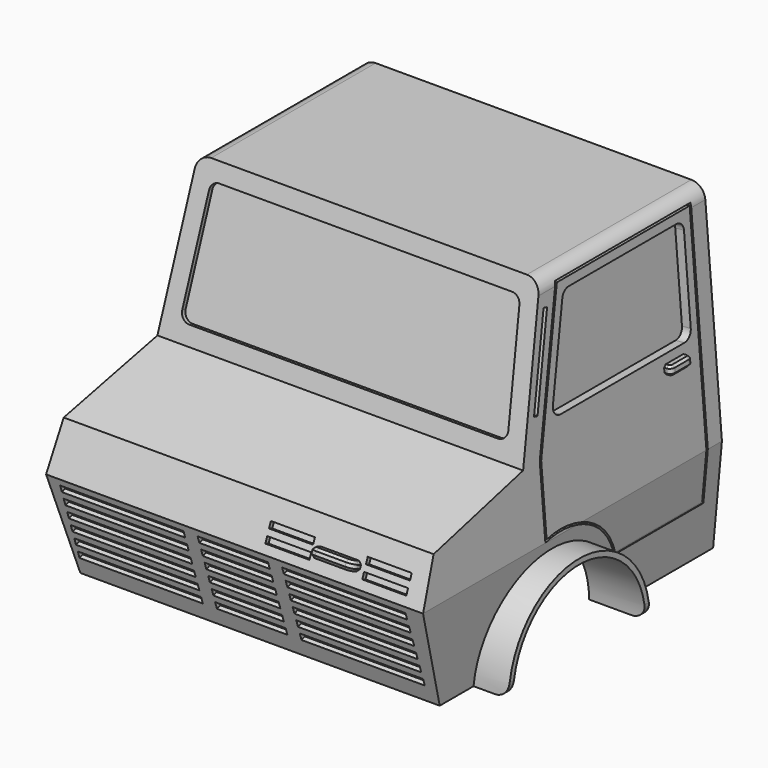
from build123d import *

# Parameters (mm, degrees)
F1_DEPTH       = 2140
F3_DEPTH       = 2500
F4_W           = 400
F4_H           = 40
F4_W_2         = 700
F5_DEPTH       = 25
F7_DEPTH       = 25
F9_DEPTH       = 50
F11_DEPTH      = 50
F13_DEPTH      = 150
F13_DEPTH_BACK = 2290
F14_T1_DEPTH   = 430
F14_T3_DEPTH   = 430
F14_T8_DEPTH   = 1536.0313143724
F14_T13_DEPTH  = 1536.0313143724
F14_T18_DEPTH  = 1536.0313143724
F14_T23_DEPTH  = 1536.0313143724
F14_T28_DEPTH  = 1536.0313143724
F14_T33_DEPTH  = 1536.0313143724
F15_W          = 1800
F15_H          = 1110
F15_H_2        = 10
F15_H_3        = 730
F16_DEPTH      = 200
F18_DEPTH      = 25
F19_W          = 150
F19_H          = 50
F20_DEPTH      = 40
F21_W          = 150
F21_H          = 50
F22_DEPTH      = 40
F23_R          = 25
F24_SIZE       = 12.5
F27_DEPTH      = 25
F28_W          = 250
F28_H          = 35
F29_DEPTH      = 25
F28_H_2        = 50
F30_DEPTH      = 60
F31_R          = 40
F32_SIZE       = 15
F33_DEPTH      = 25


# Not quite as in the source:
# - a fillet or chamfer that OpenCascade refuses, or shapes differently, is made with other operations: its cross-section is extruded or revolved along the edge and cut away or added
# - a feature names something its author has since deleted; it is built from what else it names


with BuildPart() as f1:
    # F0 (on Right) → F1 (new body)
    with BuildSketch(Plane.YZ):
        with BuildLine():
            Line((-868.0252010454, -338.8581766918), (-687.2093945233, -888.8581766918))
            Line((-687.2093945233, -888.8581766918), (-447.2093945233, -888.8581766918))
            ThreePointArc((-447.2093945233, -888.8581766918), (52.7906054767, -388.8581766918), (552.7906054767, -888.8581766918))
            Line((552.7906054767, -888.8581766918), (1252.7906054767, -888.8581766918))
            Line((1252.7906054767, -888.8581766918), (1252.7906054767, 911.1418233082))
            Line((1252.7906054767, 911.1418233082), (86.0372496318, 911.1418233082))
            Line((86.0372496318, 911.1418233082), (-118.0252010454, 61.1418233082))
            Line((-118.0252010454, 61.1418233082), (-768.0252010454, -88.8581766918))
            Line((-768.0252010454, -88.8581766918), (-868.0252010454, -338.8581766918))
        make_face()
    extrude(amount=F1_DEPTH)

    # F2 (on face) → F3 (cut)
    with BuildSketch(Plane(origin=(0, 1252.7906054767, 0), x_dir=(-1, 0, 0), z_dir=(0, 1, 0))):
        Polygon((-2140, 911.1418233082), (-2140, -338.8581766918), (-2040, 911.1418233082), align=None)
        Polygon((-2140, -338.8581766918), (-2140, -888.8581766918), (-2090, -888.8581766918), align=None)
        Polygon((0, -338.8581766918), (-50, -888.8581766918), (0, -888.8581766918), align=None)
        Polygon((-100, 911.1418233082), (0, -338.8581766918), (0, 911.1418233082), align=None)
    extrude(amount=-F3_DEPTH, mode=Mode.SUBTRACT)

    # F4 (on face) → F5 (cut)
    with BuildSketch(Plane(origin=(0, -883.8950331202, -290.5858059899), x_dir=(1, 0, 0), z_dir=(0, -0.9499797347, -0.3123115489))):
        with Locations((1050, -110.8141057509)):
            Rectangle(F4_W, F4_H)
        with Locations((1680, -110.8141057509)):
            Rectangle(F4_W_2, F4_H)
        with Locations((1680, -190.8141057509)):
            Rectangle(F4_W_2, F4_H)
        with Locations((1050, -190.8141057509)):
            Rectangle(F4_W, F4_H)
        with Locations((420, -190.8141057509)):
            Rectangle(F4_W_2, F4_H)
        with Locations((420, -110.8141057509)):
            Rectangle(F4_W_2, F4_H)
        with Locations((420, -270.8141057509)):
            Rectangle(F4_W_2, F4_H)
        with Locations((1050, -270.8141057509)):
            Rectangle(F4_W, F4_H)
        with Locations((1680, -270.8141057509)):
            Rectangle(F4_W_2, F4_H)
        with Locations((1680, -350.8141057509)):
            Rectangle(F4_W_2, F4_H)
        with Locations((1050, -350.8141057509)):
            Rectangle(F4_W, F4_H)
        with Locations((420, -350.8141057509)):
            Rectangle(F4_W_2, F4_H)
        with Locations((420, -430.8141057509)):
            Rectangle(F4_W_2, F4_H)
        with Locations((1050, -430.8141057509)):
            Rectangle(F4_W, F4_H)
        with Locations((1680, -430.8141057509)):
            Rectangle(F4_W_2, F4_H)
        with Locations((1050, -510.8141057509)):
            Rectangle(F4_W, F4_H)
        with Locations((1680, -510.8141057509)):
            Rectangle(F4_W_2, F4_H)
        with Locations((420, -510.8141057509)):
            Rectangle(F4_W_2, F4_H)
    extrude(amount=-F5_DEPTH, mode=Mode.SUBTRACT)

    # F6 (on face) → F7 (cut)
    with BuildSketch(Plane(origin=(0, -125.4721115769, 30.1225253883), x_dir=(1, 0, 0), z_dir=(0, -0.9723710875, 0.2334405025))):
        with BuildLine():
            ThreePointArc((238.7847050975, 806.0525443848), (204.8280302743, 792.7532832732), (188.9353028494, 759.9303137829))
            Line((188.9353028494, 759.9303137829), (144.2722089495, 185.7784483863))
            ThreePointArc((144.2722089495, 185.7784483863), (157.4208723093, 147.944004165), (194.1216111976, 131.9006789882))
            Line((194.1216111976, 131.9006789882), (1945.8783888024, 131.9006789882))
            ThreePointArc((1945.8783888024, 131.9006789882), (1982.5791276907, 147.944004165), (1995.7277910505, 185.7784483863))
            Line((1995.7277910505, 185.7784483863), (1951.0646971506, 759.9303137829))
            ThreePointArc((1951.0646971506, 759.9303137829), (1935.1719697257, 792.7532832732), (1901.2152949025, 806.0525443848))
            Line((1901.2152949025, 806.0525443848), (238.7847050975, 806.0525443848))
        make_face()
    extrude(amount=-F7_DEPTH, mode=Mode.SUBTRACT)

    # F8 (on face) → F9 (cut)
    with BuildSketch(Plane(origin=(2099.4548349212, 0, 167.9563867937), x_dir=(0, 1, 0), z_dir=(0.9968152785, 0, 0.0797452223))):
        with BuildLine():
            Line((1152.7906054767, -508.4337834687), (1152.7906054767, 695.5598369298))
            Line((1152.7906054767, 695.5598369298), (192.4028323197, 695.5598369298))
            Line((192.4028323197, 695.5598369298), (0, -108.4337834687))
            Line((0, -108.4337834687), (0, -508.4337834687))
            ThreePointArc((0, -508.4337834687), (111.5695780666, -493.7074634076), (223.1391561332, -508.4337834687))
            Line((223.1391561332, -508.4337834687), (256.9923092676, -508.4337834687))
            ThreePointArc((256.9923092676, -508.4337834687), (134.4170810173, -484.3010551602), (10, -495.5910997734))
            Line((10, -495.5910997734), (10, -109.6136704941))
            Line((10, -109.6136704941), (200.2921007484, 685.5598369298))
            Line((200.2921007484, 685.5598369298), (1142.7906054767, 685.5598369298))
            Line((1142.7906054767, 685.5598369298), (1142.7906054767, -508.4337834687))
            Line((1142.7906054767, -508.4337834687), (1152.7906054767, -508.4337834687))
        make_face()
        with BuildLine():
            Line((1152.7906054767, -782.6949255494), (1152.7906054767, -508.4337834687))
            Line((1152.7906054767, -508.4337834687), (1142.7906054767, -508.4337834687))
            Line((1142.7906054767, -508.4337834687), (1142.7906054767, -772.6949255494))
            Line((1142.7906054767, -772.6949255494), (524.8433534379, -772.6949255494))
            ThreePointArc((524.8433534379, -772.6949255494), (420.590506836, -610.4885853327), (256.9923092676, -508.4337834687))
            Line((256.9923092676, -508.4337834687), (223.1391561332, -508.4337834687))
            ThreePointArc((223.1391561332, -508.4337834687), (404.5398026813, -608.9560575502), (517.7905329259, -782.6949255494))
            Line((517.7905329259, -782.6949255494), (1152.7906054767, -782.6949255494))
        make_face()
        with BuildLine():
            ThreePointArc((1092.7906054767, 585.5598369298), (1078.145944536, 620.9151759891), (1042.7906054767, 635.5598369298))
            Line((1042.7906054767, 635.5598369298), (279.1847850354, 635.5598369298))
            ThreePointArc((279.1847850354, 635.5598369298), (248.215796316, 624.8144129394), (230.5578041703, 597.1967064375))
            Line((230.5578041703, 597.1967064375), (115.6895301314, 117.1967064375))
            ThreePointArc((115.6895301314, 117.1967064375), (125.061934987, 74.5908482103), (164.3165109966, 55.5598369298))
            Line((164.3165109966, 55.5598369298), (1042.7906054767, 55.5598369298))
            ThreePointArc((1042.7906054767, 55.5598369298), (1078.145944536, 70.2044978704), (1092.7906054767, 105.5598369298))
            Line((1092.7906054767, 105.5598369298), (1092.7906054767, 585.5598369298))
        make_face()
    extrude(amount=-F9_DEPTH, mode=Mode.SUBTRACT)

    # F10 (on face) → F11 (cut)
    with BuildSketch(Plane(origin=(26.9362620582, 0, -2.1549009647), x_dir=(0, -1, 0), z_dir=(-0.9968152785, 0, 0.0797452223))):
        with BuildLine():
            Line((-1152.7906054767, -612.040149864), (-517.7376456074, -612.040149864))
            ThreePointArc((-517.7376456074, -612.040149864), (-312.7747219376, -373.0527728554), (0.0839169816, -337.7790077833))
            Line((0.0839169816, -337.7790077833), (0.0839169816, 62.2209922167))
            Line((0.0839169816, 62.2209922167), (-192.318915338, 866.2146126152))
            Line((-192.318915338, 866.2146126152), (-1152.7906054767, 866.2146126152))
            Line((-1152.7906054767, 866.2146126152), (-1152.7906054767, -612.040149864))
        make_face()
        with BuildLine():
            Line((-1142.7906054767, -602.040149864), (-1142.7906054767, 856.2146126152))
            Line((-1142.7906054767, 856.2146126152), (-200.2081837667, 856.2146126152))
            Line((-200.2081837667, 856.2146126152), (-9.9160830184, 61.0411051913))
            Line((-9.9160830184, 61.0411051913), (-9.9160830184, -324.9354323363))
            ThreePointArc((-9.9160830184, -324.9354323363), (-320.0389671232, -365.5952501122), (-524.7906054767, -602.040149864))
            Line((-524.7906054767, -602.040149864), (-1142.7906054767, -602.040149864))
        make_face(mode=Mode.SUBTRACT)
        with BuildLine():
            ThreePointArc((-1042.7906054767, 806.2146126152), (-1078.145944536, 791.5699516745), (-1092.7906054767, 756.2146126152))
            Line((-1092.7906054767, 756.2146126152), (-1092.7906054767, 276.2146126152))
            ThreePointArc((-1092.7906054767, 276.2146126152), (-1078.145944536, 240.8592735558), (-1042.7906054767, 226.2146126152))
            Line((-1042.7906054767, 226.2146126152), (-164.2325940149, 226.2146126152))
            ThreePointArc((-164.2325940149, 226.2146126152), (-124.9780180054, 245.2456238957), (-115.6056131498, 287.8514821229))
            Line((-115.6056131498, 287.8514821229), (-230.4738871887, 767.8514821229))
            ThreePointArc((-230.4738871887, 767.8514821229), (-248.1318793343, 795.4691886247), (-279.1008680538, 806.2146126152))
            Line((-279.1008680538, 806.2146126152), (-1042.7906054767, 806.2146126152))
        make_face()
    extrude(amount=-F11_DEPTH, mode=Mode.SUBTRACT)

    # F12 (on Right) → F13 (join, two sides)
    with BuildSketch(Plane.YZ) as f13_sk:
        with BuildLine():
            Line((522.7906054767, -888.8581766918), (552.7906054767, -888.8581766918))
            ThreePointArc((552.7906054767, -888.8581766918), (52.7906054767, -388.8581766918), (-447.2093945233, -888.8581766918))
            Line((-447.2093945233, -888.8581766918), (-417.2093945233, -888.8581766918))
            ThreePointArc((-417.2093945233, -888.8581766918), (52.7906054767, -418.8581773039), (522.7906054767, -888.8581766918))
        make_face()
    extrude(amount=-F13_DEPTH)
    extrude(f13_sk.sketch, amount=F13_DEPTH_BACK)

    # F14: fillet of radius 80 on 6 edges, made by hand

    # F14_s2 → F14_t1 (cut)
    with BuildSketch(Plane.XZ.offset(217.2093945233)):
        with BuildLine():
            ThreePointArc((-70, -888.8581766918), (-126.5685424949, -865.4267191867), (-150, -808.8581766918))
            Line((-150, -808.8581766918), (-150, -888.8581766918))
            Line((-150, -888.8581766918), (-70, -888.8581766918))
        make_face()
        with BuildLine():
            ThreePointArc((2210, -888.8581766918), (2266.5685424949, -865.4267191867), (2290, -808.8581766918))
            Line((2290, -808.8581766918), (2290, -888.8581766918))
            Line((2290, -888.8581766918), (2210, -888.8581766918))
        make_face()
    extrude(amount=F14_T1_DEPTH, mode=Mode.SUBTRACT)

    # F14_s4 → F14_t3 (cut)
    with BuildSketch(Plane.XZ.offset(-752.7906054767)):
        with BuildLine():
            ThreePointArc((-150, -808.8581766918), (-126.5685424949, -865.4267191867), (-70, -888.8581766918))
            Line((-70, -888.8581766918), (-150, -888.8581766918))
            Line((-150, -888.8581766918), (-150, -808.8581766918))
        make_face()
        with BuildLine():
            ThreePointArc((2290, -808.8581766918), (2266.5685424949, -865.4267191867), (2210, -888.8581766918))
            Line((2210, -888.8581766918), (2290, -888.8581766918))
            Line((2290, -888.8581766918), (2290, -808.8581766918))
        make_face()
    extrude(amount=F14_T3_DEPTH, mode=Mode.SUBTRACT)


with BuildPart() as f14_tool6:
    # F14_s7 → F14_t8 (new body)
    with BuildSketch(Plane.XZ.offset(-1437.4295847404)):
        with BuildLine():
            ThreePointArc((2045.8896305774, 837.5214410908), (2020.4105606244, 889.9226425548), (1966.1444082945, 911.1418233082))
            Line((1966.1444082945, 911.1418233082), (2040, 911.1418233082))
            Line((2040, 911.1418233082), (2045.8896305774, 837.5214410908))
        make_face()
    extrude(amount=F14_T8_DEPTH)

    split(bisect_by=Plane.XZ.offset(-1142.7906054767), keep=Keep.BOTTOM)


with BuildPart() as f1_1:
    add(f1.part)

    # F14_t5: cut F14_tool6
    add(f14_tool6.part, mode=Mode.SUBTRACT)


with BuildPart() as f14_tool11:
    # F14_s12 → F14_t13 (new body)
    with BuildSketch(Plane.XZ.offset(-1437.4295847404)):
        with BuildLine():
            ThreePointArc((2045.8896305774, 837.5214410908), (2020.4105606244, 889.9226425548), (1966.1444082945, 911.1418233082))
            Line((1966.1444082945, 911.1418233082), (2040, 911.1418233082))
            Line((2040, 911.1418233082), (2045.8896305774, 837.5214410908))
        make_face()
    extrude(amount=F14_T13_DEPTH)

    split(bisect_by=Plane(origin=(-54.6701215842, 0, 683.3765198023), x_dir=(0, 1, 0), z_dir=(-0.0797452223, 0, 0.9968152785)), keep=Keep.TOP)


with BuildPart() as f1_2:
    add(f1_1.part)

    # F14_t10: cut F14_tool11
    add(f14_tool11.part, mode=Mode.SUBTRACT)


with BuildPart() as f14_tool16:
    # F14_s17 → F14_t18 (new body)
    with BuildSketch(Plane.XZ.offset(-1437.4295847404)):
        with BuildLine():
            ThreePointArc((2045.8896305774, 837.5214410908), (2020.4105606244, 889.9226425548), (1966.1444082945, 911.1418233082))
            Line((1966.1444082945, 911.1418233082), (2040, 911.1418233082))
            Line((2040, 911.1418233082), (2045.8896305774, 837.5214410908))
        make_face()
    extrude(amount=F14_T18_DEPTH)

    split(bisect_by=Plane(origin=(0.6539804672, 34.2689853643, -8.1747558399), x_dir=(0.9998179551, -0.0190802677, 0), z_dir=(-0.0185596949, -0.9725396173, 0.2319961864)), keep=Keep.TOP)


with BuildPart() as f1_3:
    add(f1_2.part)

    # F14_t15: cut F14_tool16
    add(f14_tool16.part, mode=Mode.SUBTRACT)


with BuildPart() as f14_tool21:
    # F14_s22 → F14_t23 (new body)
    with BuildSketch(Plane.XZ.offset(-1437.4295847404)):
        with BuildLine():
            ThreePointArc((94.1103694226, 837.5214410908), (119.5894393756, 889.9226425548), (173.8555917055, 911.1418233082))
            Line((173.8555917055, 911.1418233082), (100, 911.1418233082))
            Line((100, 911.1418233082), (94.1103694226, 837.5214410908))
        make_face()
    extrude(amount=F14_T23_DEPTH)

    split(bisect_by=Plane.XZ.offset(-1142.7906054767), keep=Keep.BOTTOM)


with BuildPart() as f1_4:
    add(f1_3.part)

    # F14_t20: cut F14_tool21
    add(f14_tool21.part, mode=Mode.SUBTRACT)


with BuildPart() as f14_tool26:
    # F14_s27 → F14_t28 (new body)
    with BuildSketch(Plane.XZ.offset(-1437.4295847404)):
        with BuildLine():
            ThreePointArc((94.1103694226, 837.5214410908), (119.5894393756, 889.9226425548), (173.8555917055, 911.1418233082))
            Line((173.8555917055, 911.1418233082), (100, 911.1418233082))
            Line((100, 911.1418233082), (94.1103694226, 837.5214410908))
        make_face()
    extrude(amount=F14_T28_DEPTH)

    split(bisect_by=Plane(origin=(68.2790246049, 0, 853.4878075607), x_dir=(0, 1, 0), z_dir=(0.0797452223, 0, 0.9968152785)), keep=Keep.TOP)


with BuildPart() as f1_5:
    add(f1_4.part)

    # F14_t25: cut F14_tool26
    add(f14_tool26.part, mode=Mode.SUBTRACT)


with BuildPart() as f14_tool31:
    # F14_s32 → F14_t33 (new body)
    with BuildSketch(Plane.XZ.offset(-1437.4295847404)):
        with BuildLine():
            ThreePointArc((94.1103694226, 837.5214410908), (119.5894393756, 889.9226425548), (173.8555917055, 911.1418233082))
            Line((173.8555917055, 911.1418233082), (100, 911.1418233082))
            Line((100, 911.1418233082), (94.1103694226, 837.5214410908))
        make_face()
    extrude(amount=F14_T33_DEPTH)

    split(bisect_by=Plane(origin=(0.0846835065, -4.4374686868, 1.0585438313), x_dir=(0.9998179551, 0.0190802677, 0), z_dir=(0.0185596949, -0.9725396173, 0.2319961864)), keep=Keep.TOP)


with BuildPart() as f1_6:
    add(f1_5.part)

    # F14_t30: cut F14_tool31
    add(f14_tool31.part, mode=Mode.SUBTRACT)

    # F15 (on face) → F16 (cut)
    with BuildSketch(Plane(origin=(0, 0, -888.8581766918), x_dir=(1, 0, 0), z_dir=(0, 0, -1))):
        with Locations((1070, 32.2093945233)):
            Rectangle(F15_W, F15_H)
        with Locations((1070, -1257.7906054767)):
            Rectangle(F15_W, F15_H_2)
        with Locations((1070, -887.7906054767)):
            Rectangle(F15_W, F15_H_3)
    extrude(amount=-F16_DEPTH, mode=Mode.SUBTRACT)

    # F17 (on face) → F18 (cut)
    with BuildSketch(Plane(origin=(0, 1252.7906054767, 0), x_dir=(-1, 0, 0), z_dir=(0, 1, 0))):
        with BuildLine():
            Line((-238.4792344478, 811.1418233082), (-1901.5207655522, 811.1418233082))
            ThreePointArc((-1901.5207655522, 811.1418233082), (-1935.4371107584, 797.8798353373), (-1951.361529479, 765.1290844223))
            Line((-1951.361529479, 765.1290844223), (-1989.761529479, 285.1290844223))
            ThreePointArc((-1989.761529479, 285.1290844223), (-1976.6587775813, 247.225478102), (-1939.9207655522, 231.1418233082))
            Line((-1939.9207655522, 231.1418233082), (-200.0792344478, 231.1418233082))
            ThreePointArc((-200.0792344478, 231.1418233082), (-163.3412224187, 247.225478102), (-150.238470521, 285.1290844223))
            Line((-150.238470521, 285.1290844223), (-188.638470521, 765.1290844223))
            ThreePointArc((-188.638470521, 765.1290844223), (-204.5628892416, 797.8798353373), (-238.4792344478, 811.1418233082))
        make_face()
    extrude(amount=-F18_DEPTH, mode=Mode.SUBTRACT)

    # F19 (on face) → F20 (join)
    with BuildSketch(Plane(origin=(2099.4548349212, 0, 167.9563867937), x_dir=(0, 1, 0), z_dir=(0.9968152785, 0, 0.0797452223))):
        with Locations((967.7906054767, -19.4401630702)):
            Rectangle(F19_W, F19_H)
    extrude(amount=F20_DEPTH)

    # F21 (on face) → F22 (join)
    with BuildSketch(Plane(origin=(26.9362620582, 0, -2.1549009647), x_dir=(0, -1, 0), z_dir=(-0.9968152785, 0, 0.0797452223))):
        with Locations((-967.7906054767, 151.2146126152)):
            Rectangle(F21_W, F21_H)
    extrude(amount=F22_DEPTH)

    # F23
    f23_edges = [f1_6.edges().sort_by_distance(p)[0] for p in [
        (2140.877706, 1042.790605, 151.767944),
        (2140.877706, 892.790605, 151.767944),
        (-0.877706, 892.790605, 151.767944),
        (-0.877706, 1042.790605, 151.767944),
    ]]
    fillet(f23_edges, radius=F23_R)

    # F24
    f24_edges = [f1_6.edges().sort_by_distance(p)[0] for p in [
        (2106.487579, 1042.790605, 174.096606),
        (2142.871337, 967.790605, 126.847562),
        (1.115924, 967.790605, 176.688326),
        (-2.871337, 967.790605, 126.847562),
        (29.52516, 892.790605, 124.255842),
        (33.512421, 892.790605, 174.096606),
        (29.52516, 1042.790605, 124.255842),
        (4.427674, 1035.468275, 126.263641),
        (4.427674, 900.112936, 126.263641),
        (8.414935, 900.112936, 176.104405),
        (33.512421, 1042.790605, 174.096606),
        (8.414935, 1035.468275, 176.104405),
        (2106.487579, 892.790605, 174.096606),
        (2110.47484, 892.790605, 124.255842),
        (2131.585065, 1035.468275, 176.104405),
        (2138.884076, 967.790605, 176.688326),
        (2131.585065, 900.112936, 176.104405),
        (2110.47484, 1042.790605, 124.255842),
        (2135.572326, 900.112936, 126.263641),
        (2135.572326, 1035.468275, 126.263641),
    ]]
    chamfer(f24_edges, length=F24_SIZE)

    # F25 (on face) → F27 (cut)
    with BuildSketch(Plane(origin=(2099.4548349212, 0, 167.9563867937), x_dir=(0, 1, 0), z_dir=(0.9968152785, 0, 0.0797452223))):
        Polygon((122.1902180749, 595.8640537001), (97.8767276423, 601.682488454), (-18.4919674348, 115.4126798024), (5.8215229978, 109.5942450485), align=None)
    extrude(amount=-F27_DEPTH, mode=Mode.SUBTRACT)

    # F28 (on face) → F29 (cut)
    with BuildSketch(Plane(origin=(0, -631.449939973, 252.5799759892), x_dir=(1, 0, 0), z_dir=(0, -0.9284766909, 0.3713906764))):
        with Locations((1905, -569.4983850829)):
            Rectangle(F28_W, F28_H)
        with Locations((1905, -499.4983850829)):
            Rectangle(F28_W, F28_H)
        with Locations((1355, -499.4983850829)):
            Rectangle(F28_W, F28_H)
        with Locations((1355, -569.4983850829)):
            Rectangle(F28_W, F28_H)
    extrude(amount=-F29_DEPTH, mode=Mode.SUBTRACT)

    # F28 (on face) → F30 (join)
    with BuildSketch(Plane(origin=(0, -631.449939973, 252.5799759892), x_dir=(1, 0, 0), z_dir=(0, -0.9284766909, 0.3713906764))):
        with Locations((1630, -536.9983850829)):
            Rectangle(F28_W, F28_H_2)
    extrude(amount=F30_DEPTH)

    # F31
    f31_edges = [f1_6.edges().sort_by_distance(p)[0] for p in [
        (1755, -886.594735, -223.727067),
        (1505, -886.594735, -223.727067),
    ]]
    fillet(f31_edges, radius=F31_R)

    # F32
    f32_edges = [f1_6.edges().sort_by_distance(p)[0] for p in [
        (1630, -895.879502, -246.938984),
        (1630, -877.309968, -200.51515),
        (1755, -849.455667, -265.508518),
        (1755, -830.886133, -219.084684),
        (1505, -849.455667, -265.508518),
        (1516.715729, -885.001721, -251.290097),
        (1743.284271, -885.001721, -251.290097),
        (1743.284271, -866.432187, -204.866262),
        (1505, -830.886133, -219.084684),
        (1516.715729, -866.432187, -204.866262),
    ]]
    chamfer(f32_edges, length=F32_SIZE)

    # F26 (on face) → F33 (cut)
    with BuildSketch(Plane(origin=(26.9362620582, 0, -2.1549009647), x_dir=(0, -1, 0), z_dir=(-0.9968152785, 0, 0.0797452223))):
        Polygon((18.4942401875, 286.0579583373), (-97.8744548896, 772.3277669888), (-122.1879453222, 766.509332235), (-5.8192502451, 280.2395235834), align=None)
    extrude(amount=-F33_DEPTH, mode=Mode.SUBTRACT)


solid = f1_6.part
